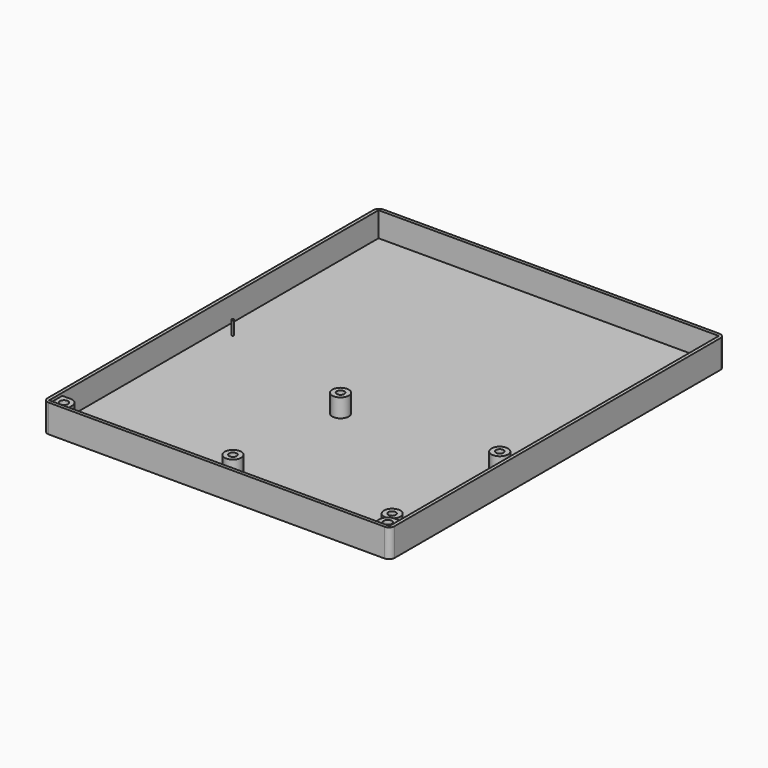
from build123d import *

# Parameters (mm, degrees)
F0_W           = 126.4
F0_H           = 152.4
F0_W_2         = 124
F0_H_2         = 150
F1_DEPTH       = 10.2
F2_DEPTH       = 1.2
F3_R           = 2
F4_R           = 1.5
F5_DEPTH       = 9.2
F6_D           = 3
F6_CBORE_D     = 4
F6_CBORE_DEPTH = 1.2
F7_R           = 3
F7_R_2         = 1.375
F8_DEPTH       = 6.7
F7_R_3         = 0.4
F9_DEPTH       = 5


# Not quite as in the source:
# - a feature names something its author has since deleted; it is built from what else it names


with BuildPart() as f1:
    # F0 (on Top) → F1 (new body)
    with BuildSketch(Plane.XY):
        Rectangle(F0_W, F0_H)
        Rectangle(F0_W_2, F0_H_2, mode=Mode.SUBTRACT)
    extrude(amount=F1_DEPTH)

    # F0 (on Top) → F2 (join)
    with BuildSketch(Plane.XY):
        Rectangle(F0_W_2, F0_H_2)
    extrude(amount=F2_DEPTH)

    # F3
    f3_edges = [f1.edges().sort_by_distance(p)[0] for p in [
        (63.2, -76.2, 5.1),
        (-63.2, 76.2, 5.1),
        (63.2, 76.2, 5.1),
        (-63.2, -76.2, 5.1),
    ]]
    fillet(f3_edges, radius=F3_R)

    # F4 (on face) → F5 (join)
    with BuildSketch(Plane(origin=(0, 0, 0), x_dir=(1, 0, 0), z_dir=(0, 0, -1))):
        with BuildLine():
            Line((62, 69), (62, 75))
            Line((62, 75), (56, 75))
            Line((56, 75), (56, 72))
            ThreePointArc((56, 72), (56.8786796564, 69.8786796564), (59, 69))
            Line((59, 69), (62, 69))
        make_face()
        with Locations((59, 72)):
            Circle(F4_R, mode=Mode.SUBTRACT)
        with Locations((59, 72)):
            Circle(F4_R)
        with BuildLine():
            Line((-56, 75), (-62, 75))
            Line((-62, 75), (-62, 69))
            Line((-62, 69), (-59, 69))
            ThreePointArc((-59, 69), (-56.8786796564, 69.8786796564), (-56, 72))
            Line((-56, 72), (-56, 75))
        make_face()
        with Locations((-59, 72)):
            Circle(F4_R, mode=Mode.SUBTRACT)
        with Locations((-59, 72)):
            Circle(F4_R)
    extrude(amount=-F5_DEPTH)

    # F6 (through all)
    with Locations(Plane(origin=(0, 0, 0), x_dir=(1, 0, 0), z_dir=(0, 0, -1))):
        with Locations((59, 72), (-59, 72)):
            CounterBoreHole(F6_D / 2, F6_CBORE_D / 2, F6_CBORE_DEPTH)

    # F7 (on face) → F8 (join)
    with BuildSketch(Plane.XY.offset(1.2)):
        with Locations((55.0223472919, -16.0672999918)):
            Circle(F7_R)
        with Locations((55.0223472919, -16.0672999918)):
            Circle(F7_R_2, mode=Mode.SUBTRACT)
        with Locations((-2.9776527081, -16.0672999918)):
            Circle(F7_R)
        with Locations((-2.9776527081, -16.0672999918)):
            Circle(F7_R_2, mode=Mode.SUBTRACT)
        with Locations((-2.9776527081, -65.0672999918)):
            Circle(F7_R)
        with Locations((-2.9776527081, -65.0672999918)):
            Circle(F7_R_2, mode=Mode.SUBTRACT)
        with Locations((55.0223472919, -65.0672999918)):
            Circle(F7_R)
        with Locations((55.0223472919, -65.0672999918)):
            Circle(F7_R_2, mode=Mode.SUBTRACT)
    extrude(amount=F8_DEPTH)

    # F7 (on face) → F9 (join)
    with BuildSketch(Plane.XY.offset(1.2)):
        with Locations((-57.0500735752, 2.4133773954)):
            Circle(F7_R_3)
    extrude(amount=F9_DEPTH)


solid = f1.part
